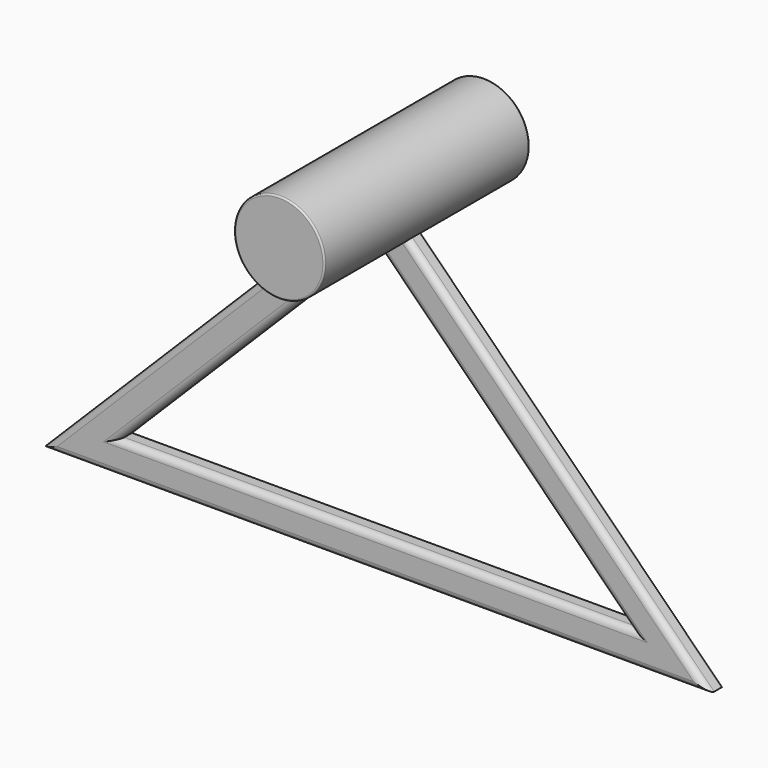
from build123d import *

# Parameters (mm, degrees)
F1_R         = 140.9846966486
F2_DEPTH     = 400
F3_DEPTH     = 25
F4_T1_DEPTH  = 2182.8427124746
F4_T6_DEPTH  = 1431.9836481951
F4_S7_R      = 140.9846966486
F4_T8_DEPTH  = 728
F4_T12_DEPTH = 1181.3708498985
F4_S13_R     = 140.9846966486
F4_T14_DEPTH = 602
F4_T19_DEPTH = 1431.9836481951
F4_S20_R     = 140.9846966486
F4_T21_DEPTH = 728
F4_T25_DEPTH = 1700
F4_T31_DEPTH = 1181.3708498985
F4_S32_R     = 140.9846966486
F4_T33_DEPTH = 602
F4_T38_DEPTH = 1181.3708498985
F4_S39_R     = 140.9846966486
F4_T40_DEPTH = 602
F4_T45_DEPTH = 1431.9836481951
F4_S46_R     = 140.9846966486
F4_T47_DEPTH = 728
F4_T52_DEPTH = 1700
F4_T56_DEPTH = 1181.3708498985
F4_T63_DEPTH = 1231.3708498985
F4_S64_R     = 140.9846966486
F4_T65_DEPTH = 627
F4_T69_DEPTH = 1231.3708498985
F4_S70_R     = 140.9846966486
F4_T71_DEPTH = 627
F4_T78_DEPTH = 1700
F4_T82_DEPTH = 1181.3708498985
F5_R         = 5


# Not quite as in the source:
# - a fillet or chamfer that OpenCascade refuses, or shapes differently, is made with other operations: its cross-section is extruded or revolved along the edge and cut away or added


with BuildPart() as f2:
    # F1 (on face) → F2 (new body, symmetric)
    with BuildSketch(Plane.XZ):
        with Locations((0, 941.6702985764)):
            Circle(F1_R)
    extrude(amount=F2_DEPTH, both=True)

    # F0 (on Front) → F3 (join, symmetric)
    with BuildSketch(Plane.XZ):
        Polygon((0, -100), (1041.4213562373, -100), (0, 941.4213562373), (-1041.4213562373, -100), align=None)
        Polygon((800, 0), (0, 0), (-800, 0), (0, 800), align=None, mode=Mode.SUBTRACT)
    extrude(amount=F3_DEPTH, both=True)

    # F4: fillet of radius 20 on 8 edges, made by hand

    # F4_s2 → F4_t1 (cut)
    with BuildSketch(Plane.YZ.offset(-1091.4213562373)):
        with BuildLine():
            ThreePointArc((-25, -80), (-19.1421356237, -94.1421356237), (-5, -100))
            Line((-5, -100), (-25, -100))
            Line((-25, -100), (-25, -80))
        make_face()
    extrude(amount=F4_T1_DEPTH, mode=Mode.SUBTRACT)


with BuildPart() as f4_tool4:
    # F4_s5 → F4_t6 (new body)
    with BuildSketch(Plane(origin=(406.4993310091, 0, 406.4993310091), x_dir=(0, 1, 0), z_dir=(-0.7071067812, 0, -0.7071067812))):
        with BuildLine():
            ThreePointArc((-25, -645.6854249492), (-19.1421356237, -659.827560573), (-5, -665.6854249492))
            Line((-5, -665.6854249492), (-25, -665.6854249492))
            Line((-25, -665.6854249492), (-25, -645.6854249492))
        make_face()
    extrude(amount=F4_T6_DEPTH)

    # F4_s7 → F4_t8 (cut, symmetric)
    with BuildSketch(Plane.XZ.offset(15)):
        with Locations((0, 941.6702985764)):
            Circle(F4_S7_R)
    extrude(amount=F4_T8_DEPTH, both=True, mode=Mode.SUBTRACT)


with BuildPart() as f2_1:
    add(f2.part)

    # F4_t3: cut F4_tool4
    add(f4_tool4.part, mode=Mode.SUBTRACT)


with BuildPart() as f4_tool10:
    # F4_s11 → F4_t12 (new body)
    with BuildSketch(Plane(origin=(-435.3553390593, 0, -435.3553390593), x_dir=(0, 1, 0), z_dir=(0.7071067812, 0, 0.7071067812))):
        with BuildLine():
            ThreePointArc((-25, 585.6854249492), (-19.1421356237, 571.5432893255), (-5, 565.6854249492))
            Line((-5, 565.6854249492), (-25, 565.6854249492))
            Line((-25, 565.6854249492), (-25, 585.6854249492))
        make_face()
    extrude(amount=F4_T12_DEPTH)

    # F4_s13 → F4_t14 (cut, symmetric)
    with BuildSketch(Plane.XZ.offset(15)):
        with Locations((0, 941.6702985764)):
            Circle(F4_S13_R)
    extrude(amount=F4_T14_DEPTH, both=True, mode=Mode.SUBTRACT)

    split(bisect_by=Plane.XY, keep=Keep.TOP)


with BuildPart() as f2_2:
    add(f2_1.part)

    # F4_t9: cut F4_tool10
    add(f4_tool10.part, mode=Mode.SUBTRACT)


with BuildPart() as f4_tool17:
    # F4_s18 → F4_t19 (new body)
    with BuildSketch(Plane(origin=(406.4993310091, 0, 406.4993310091), x_dir=(0, 1, 0), z_dir=(-0.7071067812, 0, -0.7071067812))):
        with BuildLine():
            ThreePointArc((25, -645.6854249492), (19.1421356237, -659.827560573), (5, -665.6854249492))
            Line((5, -665.6854249492), (25, -665.6854249492))
            Line((25, -665.6854249492), (25, -645.6854249492))
        make_face()
    extrude(amount=F4_T19_DEPTH)

    # F4_s20 → F4_t21 (cut, symmetric)
    with BuildSketch(Plane.XZ.offset(-15)):
        with Locations((0, 941.6702985764)):
            Circle(F4_S20_R)
    extrude(amount=F4_T21_DEPTH, both=True, mode=Mode.SUBTRACT)


with BuildPart() as f2_3:
    add(f2_2.part)

    # F4_t16: cut F4_tool17
    add(f4_tool17.part, mode=Mode.SUBTRACT)


with BuildPart() as f4_tool23:
    # F4_s24 → F4_t25 (new body)
    with BuildSketch(Plane.YZ.offset(850)):
        with BuildLine():
            ThreePointArc((-25, -20), (-19.1421356237, -5.8578643763), (-5, 0))
            Line((-5, 0), (-25, 0))
            Line((-25, 0), (-25, -20))
        make_face()
    extrude(amount=-F4_T25_DEPTH)

    split(bisect_by=Plane(origin=(-400, 0, 400), x_dir=(0, 1, 0), z_dir=(0.7071067812, 0, -0.7071067812)), keep=Keep.TOP)

    split(bisect_by=Plane(origin=(400, 0, 400), x_dir=(0, 1, 0), z_dir=(-0.7071067812, 0, -0.7071067812)), keep=Keep.TOP)


with BuildPart() as f2_4:
    add(f2_3.part)

    # F4_t22: cut F4_tool23
    add(f4_tool23.part, mode=Mode.SUBTRACT)


with BuildPart() as f4_tool29:
    # F4_s30 → F4_t31 (new body)
    with BuildSketch(Plane(origin=(-400, 0, 400), x_dir=(0, 1, 0), z_dir=(0.7071067812, 0, -0.7071067812))):
        with BuildLine():
            ThreePointArc((-25, 585.6854249492), (-19.1421356237, 571.5432893255), (-5, 565.6854249492))
            Line((-5, 565.6854249492), (-25, 565.6854249492))
            Line((-25, 565.6854249492), (-25, 585.6854249492))
        make_face()
    extrude(amount=F4_T31_DEPTH)

    # F4_s32 → F4_t33 (cut, symmetric)
    with BuildSketch(Plane.XZ.offset(15)):
        with Locations((0, 941.6702985764)):
            Circle(F4_S32_R)
    extrude(amount=F4_T33_DEPTH, both=True, mode=Mode.SUBTRACT)

    split(bisect_by=Plane.XY, keep=Keep.TOP)


with BuildPart() as f2_5:
    add(f2_4.part)

    # F4_t28: cut F4_tool29
    add(f4_tool29.part, mode=Mode.SUBTRACT)


with BuildPart() as f4_tool36:
    # F4_s37 → F4_t38 (new body)
    with BuildSketch(Plane(origin=(-400, 0, 400), x_dir=(0, 1, 0), z_dir=(0.7071067812, 0, -0.7071067812))):
        with BuildLine():
            ThreePointArc((25, 585.6854249492), (19.1421356237, 571.5432893255), (5, 565.6854249492))
            Line((5, 565.6854249492), (25, 565.6854249492))
            Line((25, 565.6854249492), (25, 585.6854249492))
        make_face()
    extrude(amount=F4_T38_DEPTH)

    # F4_s39 → F4_t40 (cut, symmetric)
    with BuildSketch(Plane.XZ.offset(-15)):
        with Locations((0, 941.6702985764)):
            Circle(F4_S39_R)
    extrude(amount=F4_T40_DEPTH, both=True, mode=Mode.SUBTRACT)

    split(bisect_by=Plane.XY, keep=Keep.TOP)


with BuildPart() as f2_6:
    add(f2_5.part)

    # F4_t35: cut F4_tool36
    add(f4_tool36.part, mode=Mode.SUBTRACT)


with BuildPart() as f4_tool43:
    # F4_s44 → F4_t45 (new body)
    with BuildSketch(Plane(origin=(606.066017178, 0, -606.066017178), x_dir=(0, 1, 0), z_dir=(-0.7071067812, 0, 0.7071067812))):
        with BuildLine():
            ThreePointArc((-5, -665.6854249492), (-19.1421356237, -659.827560573), (-25, -645.6854249492))
            Line((-25, -645.6854249492), (-25, -665.6854249492))
            Line((-25, -665.6854249492), (-5, -665.6854249492))
        make_face()
    extrude(amount=F4_T45_DEPTH)

    # F4_s46 → F4_t47 (cut, symmetric)
    with BuildSketch(Plane.XZ.offset(15)):
        with Locations((0, 941.6702985764)):
            Circle(F4_S46_R)
    extrude(amount=F4_T47_DEPTH, both=True, mode=Mode.SUBTRACT)


with BuildPart() as f2_7:
    add(f2_6.part)

    # F4_t42: cut F4_tool43
    add(f4_tool43.part, mode=Mode.SUBTRACT)


with BuildPart() as f4_tool50:
    # F4_s51 → F4_t52 (new body)
    with BuildSketch(Plane.YZ.offset(850)):
        with BuildLine():
            ThreePointArc((-25, -20), (-19.1421356237, -5.8578643763), (-5, 0))
            Line((-5, 0), (-25, 0))
            Line((-25, 0), (-25, -20))
        make_face()
    extrude(amount=-F4_T52_DEPTH)

    split(bisect_by=Plane(origin=(-400, 0, 400), x_dir=(0, 1, 0), z_dir=(-0.7071067812, 0, 0.7071067812)), keep=Keep.TOP)


with BuildPart() as f4_tool54:
    # F4_s55 → F4_t56 (new body)
    with BuildSketch(Plane(origin=(-435.3553390593, 0, -435.3553390593), x_dir=(0, 1, 0), z_dir=(0.7071067812, 0, 0.7071067812))):
        with BuildLine():
            ThreePointArc((-25, 585.6854249492), (-19.1421356237, 571.5432893255), (-5, 565.6854249492))
            Line((-5, 565.6854249492), (-25, 565.6854249492))
            Line((-25, 565.6854249492), (-25, 585.6854249492))
        make_face()
    extrude(amount=F4_T56_DEPTH)

    split(bisect_by=Plane.XY, keep=Keep.BOTTOM)


with BuildPart() as f4_tool50_1:
    add(f4_tool50.part)

    # F4_t58: intersect F4_tool54
    add(f4_tool54.part, mode=Mode.INTERSECT)


with BuildPart() as f2_8:
    add(f2_7.part)

    # F4_t48: cut F4_tool50
    add(f4_tool50_1.part, mode=Mode.SUBTRACT)


with BuildPart() as f4_tool61:
    # F4_s62 → F4_t63 (new body)
    with BuildSketch(Plane(origin=(-435.3553390593, 0, 435.3553390593), x_dir=(0, 1, 0), z_dir=(0.7071067812, 0, -0.7071067812))):
        with BuildLine():
            ThreePointArc((-25, 585.6854249492), (-19.1421356237, 571.5432893255), (-5, 565.6854249492))
            Line((-5, 565.6854249492), (-25, 565.6854249492))
            Line((-25, 565.6854249492), (-25, 585.6854249492))
        make_face()
    extrude(amount=F4_T63_DEPTH)

    # F4_s64 → F4_t65 (cut, symmetric)
    with BuildSketch(Plane.XZ.offset(15)):
        with Locations((0, 941.6702985764)):
            Circle(F4_S64_R)
    extrude(amount=F4_T65_DEPTH, both=True, mode=Mode.SUBTRACT)

    split(bisect_by=Plane(origin=(-400, 0, 400), x_dir=(0, 1, 0), z_dir=(-0.7071067812, 0, 0.7071067812)), keep=Keep.TOP)


with BuildPart() as f4_tool67:
    # F4_s68 → F4_t69 (new body)
    with BuildSketch(Plane(origin=(-435.3553390593, 0, -435.3553390593), x_dir=(0, 1, 0), z_dir=(0.7071067812, 0, 0.7071067812))):
        with BuildLine():
            ThreePointArc((-25, 585.6854249492), (-19.1421356237, 571.5432893255), (-5, 565.6854249492))
            Line((-5, 565.6854249492), (-25, 565.6854249492))
            Line((-25, 565.6854249492), (-25, 585.6854249492))
        make_face()
    extrude(amount=F4_T69_DEPTH)

    # F4_s70 → F4_t71 (cut, symmetric)
    with BuildSketch(Plane.XZ.offset(15)):
        with Locations((0, 941.6702985764)):
            Circle(F4_S70_R)
    extrude(amount=F4_T71_DEPTH, both=True, mode=Mode.SUBTRACT)

    split(bisect_by=Plane(origin=(400, 0, 400), x_dir=(0, 1, 0), z_dir=(0.7071067812, 0, 0.7071067812)), keep=Keep.TOP)


with BuildPart() as f4_tool61_1:
    add(f4_tool61.part)

    # F4_t73: intersect F4_tool67
    add(f4_tool67.part, mode=Mode.INTERSECT)


with BuildPart() as f2_9:
    add(f2_8.part)

    # F4_t59: cut F4_tool61
    add(f4_tool61_1.part, mode=Mode.SUBTRACT)


with BuildPart() as f4_tool76:
    # F4_s77 → F4_t78 (new body)
    with BuildSketch(Plane.YZ.offset(850)):
        with BuildLine():
            ThreePointArc((-25, -20), (-19.1421356237, -5.8578643763), (-5, 0))
            Line((-5, 0), (-25, 0))
            Line((-25, 0), (-25, -20))
        make_face()
    extrude(amount=-F4_T78_DEPTH)

    split(bisect_by=Plane(origin=(400, 0, 400), x_dir=(0, 1, 0), z_dir=(0.7071067812, 0, 0.7071067812)), keep=Keep.TOP)


with BuildPart() as f4_tool80:
    # F4_s81 → F4_t82 (new body)
    with BuildSketch(Plane(origin=(-400, 0, 400), x_dir=(0, 1, 0), z_dir=(0.7071067812, 0, -0.7071067812))):
        with BuildLine():
            ThreePointArc((-25, 585.6854249492), (-19.1421356237, 571.5432893255), (-5, 565.6854249492))
            Line((-5, 565.6854249492), (-25, 565.6854249492))
            Line((-25, 565.6854249492), (-25, 585.6854249492))
        make_face()
    extrude(amount=F4_T82_DEPTH)

    split(bisect_by=Plane.XY, keep=Keep.BOTTOM)


with BuildPart() as f4_tool76_1:
    add(f4_tool76.part)

    # F4_t84: intersect F4_tool80
    add(f4_tool80.part, mode=Mode.INTERSECT)


with BuildPart() as f2_10:
    add(f2_9.part)

    # F4_t74: cut F4_tool76
    add(f4_tool76_1.part, mode=Mode.SUBTRACT)

    # F5
    f5_edges = [f2_10.edges().sort_by_distance(p)[0] for p in [
        (-140.984697, 400, 941.670299),
        (-140.984697, -400, 941.670299),
    ]]
    fillet(f5_edges, radius=F5_R)


solid = f2_10.part
